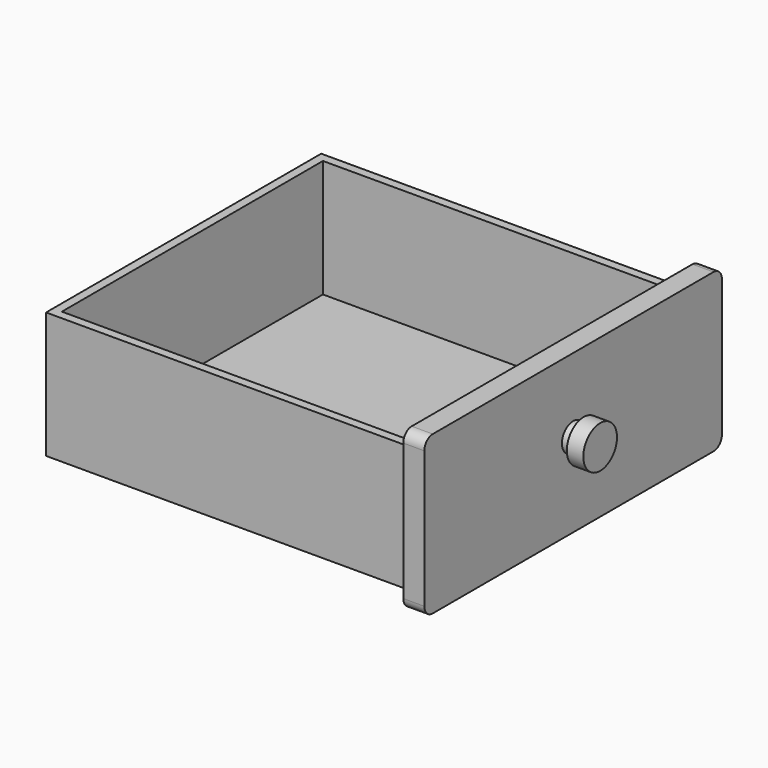
from build123d import *

# Parameters (mm, degrees)
F0_W        = 105
F0_H        = 98
F1_DEPTH    = 36
F2_DEPTH    = 42
F3_DEPTH    = 3
F4_T        = 2.5
F4_T3_DEPTH = 41
F4_T5_DEPTH = 103
F5_R        = 3
F6_R        = 4
F7_DEPTH    = 3
F8_R        = 6
F9_DEPTH    = 4.7


# Not quite as in the source:
# - a shell that OpenCascade refuses in one call is made with other operations: the cavity is built on its own and cut out


with BuildPart() as f1:
    # F0 (on Top) → F1 (new body)
    with BuildSketch(Plane.XY):
        with Locations((52.5, 0)):
            Rectangle(F0_W, F0_H)
    extrude(amount=F1_DEPTH)

    # F0 (on Top) → F2 (join)
    with BuildSketch(Plane.XY):
        Polygon((105, 53), (105, 49), (105, -49), (105, -53), (111, -53), (111, 53), align=None)
    extrude(amount=F2_DEPTH)

    # F0 (on Top) → F3 (join)
    with BuildSketch(Plane.XY):
        Polygon((105, 53), (105, 49), (105, -49), (105, -53), (111, -53), (111, 53), align=None)
    extrude(amount=-F3_DEPTH)

    # F4: shell of thickness 2.5, made by hand


with BuildPart() as f4_core1:
    # F4_t2: copy of F1
    add(f1.part)

    # the walls: a layer under each face that stays
    f4_faces = [f4_core1.faces().sort_by_distance(p)[0] for p in [
        (105, 45.4285714286, 38.7857142857),
        (108, 0, 42),
        (111, 0, 19.5),
        (108, 53, 19.5),
        (108, 0, -3),
        (108, -53, 19.5),
        (0, 0, 18),
        (52.5, -49, 18),
        (52.5, 0, 0),
        (52.5, 49, 18),
    ]]
    thicken(f4_faces, amount=-F4_T, mode=Mode.SUBTRACT)

    # F4_s4 → F4_t3 (cut)
    with BuildSketch(Plane.XY.offset(-2.5)):
        Polygon((104.975, 49.025), (107.5, 49), (107.5, 46.5), (105, 46.5), align=None)
        Polygon((104.975, -49.025), (107.5, -49), (107.5, -46.5), (105, -46.5), align=None)
    extrude(amount=F4_T3_DEPTH, mode=Mode.SUBTRACT)

    # F4_s6 → F4_t5 (cut)
    with BuildSketch(Plane.XZ.offset(-51.5)):
        Polygon((104.975, -0.025), (107.5, 0), (107.5, 2.5), (105, 2.5), align=None)
    extrude(amount=F4_T5_DEPTH, mode=Mode.SUBTRACT)


with BuildPart() as f1_1:
    add(f1.part)

    # what is left inside the walls is the cavity
    f4_cavity = [f4_core1.part.solids().sort_by_distance(p)[0] for p in [
        (55, -15.5, 35.975),
    ]]
    add(f4_cavity, mode=Mode.SUBTRACT)

    # F5
    f5_edges = [f1_1.edges().sort_by_distance(p)[0] for p in [
        (108, -53, 42),
        (108, 53, 42),
        (108, 53, -3),
        (108, -53, -3),
    ]]
    fillet(f5_edges, radius=F5_R)

    # F6 (on face) → F7 (join)
    with BuildSketch(Plane.YZ.offset(111)):
        with Locations((0, 20.9335461259)):
            Circle(F6_R)
    extrude(amount=F7_DEPTH)

    # F8 (on face) → F9 (join)
    with BuildSketch(Plane.YZ.offset(114)):
        with Locations((0, 20.9335461259)):
            Circle(F8_R)
    extrude(amount=F9_DEPTH)


solid = f1_1.part
